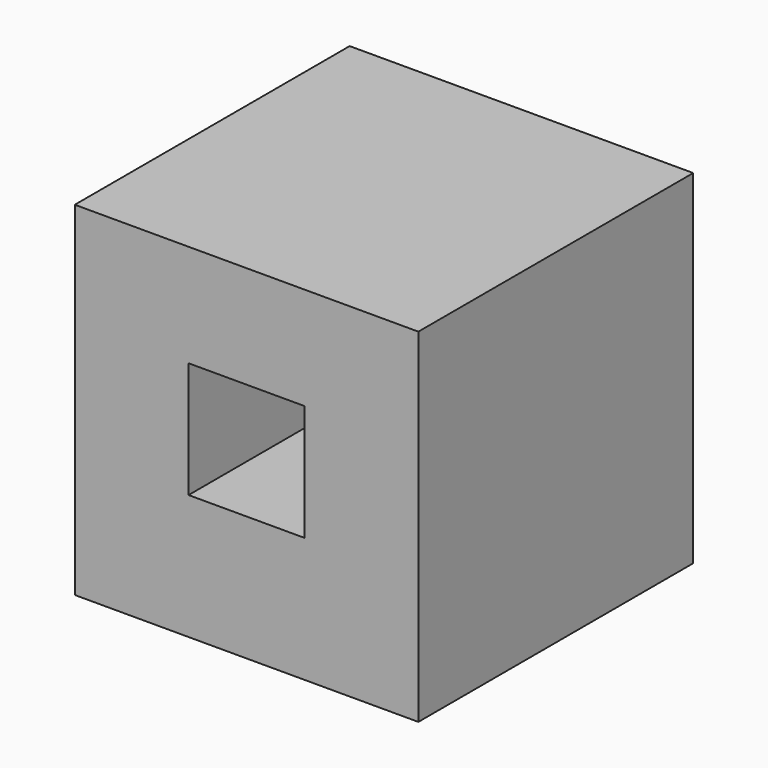
from build123d import *

# Parameters (mm, degrees)
F1_W     = 101.6
F1_H     = 101.6
F2_DEPTH = 50.8
F3_W     = 34.3186343089
F3_H     = 34.3186343089
F4_DEPTH = 46.228
F5_W     = 34.3186343089
F5_H     = 34.3186343089
F6_DEPTH = 45.974


# Not quite as in the source:
# - a variable given as a bare number and used for a length is read in inches; the dataset says mm whatever the document's units were


with BuildPart() as f2:
    # F1 (on Front) → F2 (new body, symmetric)
    with BuildSketch(Plane.XZ):
        Rectangle(F1_W, F1_H)
    extrude(amount=F2_DEPTH, both=True)

    # F3 (on face) → F4 (cut)
    with BuildSketch(Plane.XZ.offset(50.8)):
        with Locations((0, 3.3200695179)):
            Rectangle(F3_W, F3_H)
    extrude(amount=-F4_DEPTH, mode=Mode.SUBTRACT)

    # F5 (on face) → F6 (cut)
    with BuildSketch(Plane(origin=(0, 50.8, 0), x_dir=(-1, 0, 0), z_dir=(0, 1, 0))):
        with Locations((0, 3.3200695179)):
            Rectangle(F5_W, F5_H)
    extrude(amount=-F6_DEPTH, mode=Mode.SUBTRACT)


solid = f2.part
